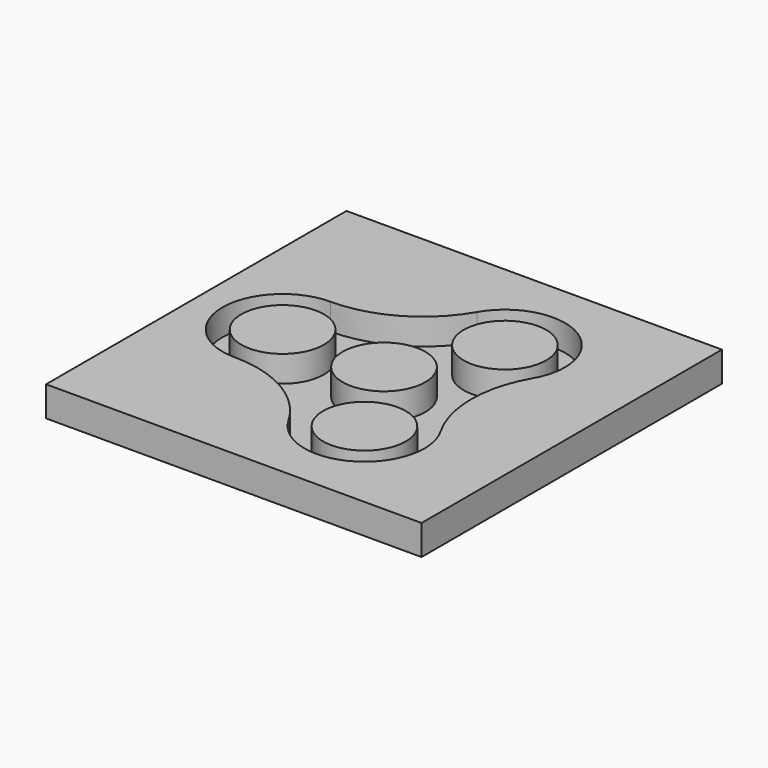
from build123d import *

# Parameters (mm, degrees)
F0_W     = 100
F0_H     = 100
F1_DEPTH = 7
F0_R     = 11
F2_DEPTH = 7
F3_R     = 3.49999
F5_W     = 100
F5_H     = 100
F6_DEPTH = 1
F7_R     = 11
F8_DEPTH = 7


# Not quite as in the source:
# - a fillet or chamfer is up to 0.001 mm smaller than in the source, because OpenCascade refuses the exact size


with BuildPart() as f1:
    # F0 (on Top) → F1 (new body)
    with BuildSketch(Plane.XY):
        Rectangle(F0_W, F0_H)
        with BuildLine():
            ThreePointArc((-27, 16), (-11.6173140978, 20.1217782649), (-0.3564064606, 31.3826859022))
            ThreePointArc((-0.3564064606, 31.3826859022), (17.6411047216, 38.8374991228), (29.5, 23.3826859022))
            ThreePointArc((29.5, 23.3826859022), (28.9548132206, 19.2415811805), (27.3564064606, 15.3826859022))
            ThreePointArc((27.3564064606, 15.3826859022), (23.2346281956, 0), (27.3564064606, -15.3826859022))
            ThreePointArc((27.3564064606, -15.3826859022), (28.9548132206, -19.2415811805), (29.5, -23.3826859022))
            ThreePointArc((29.5, -23.3826859022), (17.6411047216, -38.8374991228), (-0.3564064606, -31.3826859022))
            ThreePointArc((-0.3564064606, -31.3826859022), (-11.6173140978, -20.1217782649), (-27, -16))
            ThreePointArc((-27, -16), (-43, 0), (-27, 16))
        make_face(mode=Mode.SUBTRACT)
    extrude(amount=F1_DEPTH)


with BuildPart() as f2:
    # F0 (on Top) → F2 (new body)
    with BuildSketch(Plane.XY):
        with BuildLine():
            ThreePointArc((-16, 0), (-15.3622914957, 4.472135955), (-13.5, 8.5877820187))
            ThreePointArc((-13.5, 8.5877820187), (-19.299497169, 14.0250581514), (-27, 16))
            ThreePointArc((-27, 16), (-43, 0), (-27, -16))
            ThreePointArc((-27, -16), (-19.299497169, -14.0250581514), (-13.5, -8.5877820187))
            ThreePointArc((-13.5, -8.5877820187), (-15.3622914957, -4.472135955), (-16, 0))
        make_face()
        with Locations((-27, 0)):
            Circle(F0_R, mode=Mode.SUBTRACT)
        with BuildLine():
            ThreePointArc((-0.3564064606, 31.3826859022), (-2.4963080642, 23.7263839043), (-0.6872373903, 15.9852339604))
            ThreePointArc((-0.6872373903, 15.9852339604), (3.8081625511, 15.5402026365), (8.0000002665, 13.8564063067))
            ThreePointArc((8.0000002665, 13.8564063067), (11.5541292005, 11.068066607), (14.1872373903, 7.3974519418))
            ThreePointArc((14.1872373903, 7.3974519418), (21.7958052331, 9.7013257529), (27.3564064606, 15.3826859022))
            ThreePointArc((27.3564064606, 15.3826859022), (28.9548132206, 19.2415811805), (29.5, 23.3826859022))
            ThreePointArc((29.5, 23.3826859022), (17.6411047216, 38.8374991228), (-0.3564064606, 31.3826859022))
        make_face()
        with BuildLine():
            ThreePointArc((24.5, 23.3826859022), (19.0000001332, 13.8564065375), (8.0000002665, 13.8564063067))
            ThreePointArc((8.0000002665, 13.8564063067), (7.9999998668, 32.9089652669), (24.5, 23.3826859022))
        make_face(mode=Mode.SUBTRACT)
        with BuildLine():
            ThreePointArc((-0.6872373903, 15.9852339604), (1.9458710013, 12.3146190845), (5.5000002388, 9.5262793037))
            ThreePointArc((5.5000002388, 9.5262793037), (9.6918377323, 7.8424831962), (14.1872373903, 7.3974519418))
            ThreePointArc((14.1872373903, 7.3974519418), (11.5541292005, 11.068066607), (8.0000002665, 13.8564063067))
            ThreePointArc((8.0000002665, 13.8564063067), (3.8081625511, 15.5402026365), (-0.6872373903, 15.9852339604))
        make_face()
        with BuildLine():
            ThreePointArc((27.3564064606, -15.3826859022), (21.7958052331, -9.7013257529), (14.1872373903, -7.3974519418))
            ThreePointArc((14.1872373903, -7.3974519418), (11.5541290581, -11.0680667557), (7.99999991, -13.8564065125))
            ThreePointArc((7.99999991, -13.8564065125), (3.8081623512, -15.5402026855), (-0.6872373903, -15.9852339604))
            ThreePointArc((-0.6872373903, -15.9852339604), (-2.4963080642, -23.7263839043), (-0.3564064606, -31.3826859022))
            ThreePointArc((-0.3564064606, -31.3826859022), (17.6411047216, -38.8374991228), (29.5, -23.3826859022))
            ThreePointArc((29.5, -23.3826859022), (28.9548132206, -19.2415811805), (27.3564064606, -15.3826859022))
        make_face()
        with BuildLine():
            ThreePointArc((24.5, -23.3826859022), (8.000000045, -32.9089653698), (7.99999991, -13.8564065125))
            ThreePointArc((7.99999991, -13.8564065125), (18.999999955, -13.8564064346), (24.5, -23.3826859022))
        make_face(mode=Mode.SUBTRACT)
        with BuildLine():
            ThreePointArc((14.1872373903, -7.3974519418), (9.6918376596, -7.842483214), (5.5000001093, -9.5262793785))
            ThreePointArc((5.5000001093, -9.5262793785), (1.9458709496, -12.3146191385), (-0.6872373903, -15.9852339604))
            ThreePointArc((-0.6872373903, -15.9852339604), (3.8081623512, -15.5402026855), (7.99999991, -13.8564065125))
            ThreePointArc((7.99999991, -13.8564065125), (11.5541290581, -11.0680667557), (14.1872373903, -7.3974519418))
        make_face()
        with BuildLine():
            ThreePointArc((-0.3564064606, -31.3826859022), (-2.4963080642, -23.7263839043), (-0.6872373903, -15.9852339604))
            ThreePointArc((-0.6872373903, -15.9852339604), (-8, -13.8564064606), (-13.5, -8.5877820187))
            ThreePointArc((-13.5, -8.5877820187), (-19.299497169, -14.0250581514), (-27, -16))
            ThreePointArc((-27, -16), (-11.6173140978, -20.1217782649), (-0.3564064606, -31.3826859022))
        make_face()
        with BuildLine():
            ThreePointArc((5.5000002388, 9.5262793037), (9.5262795106, 5.4999998806), (11, 0))
            ThreePointArc((11, 0), (9.5262794732, -5.4999999453), (5.5000001093, -9.5262793785))
            ThreePointArc((5.5000001093, -9.5262793785), (9.6918376596, -7.842483214), (14.1872373903, -7.3974519418))
            ThreePointArc((14.1872373903, -7.3974519418), (15.5402026731, -3.8081624017), (16, 0))
            ThreePointArc((16, 0), (15.5402026731, 3.8081624017), (14.1872373903, 7.3974519418))
            ThreePointArc((14.1872373903, 7.3974519418), (9.6918377323, 7.8424831962), (5.5000002388, 9.5262793037))
        make_face()
        with BuildLine():
            ThreePointArc((-0.6872373903, -15.9852339604), (1.9458709496, -12.3146191385), (5.5000001093, -9.5262793785))
            ThreePointArc((5.5000001093, -9.5262793785), (-5.4999999453, -9.5262794732), (-11, 0))
            ThreePointArc((-11, 0), (-11.6377085043, -4.472135955), (-13.5, -8.5877820187))
            ThreePointArc((-13.5, -8.5877820187), (-8, -13.8564064606), (-0.6872373903, -15.9852339604))
        make_face()
        with BuildLine():
            ThreePointArc((-13.5, -8.5877820187), (-11.6377085043, -4.472135955), (-11, 0))
            ThreePointArc((-11, 0), (-11.6377085043, 4.472135955), (-13.5, 8.5877820187))
            ThreePointArc((-13.5, 8.5877820187), (-15.3622914957, 4.472135955), (-16, 0))
            ThreePointArc((-16, 0), (-15.3622914957, -4.472135955), (-13.5, -8.5877820187))
        make_face()
        with BuildLine():
            ThreePointArc((-11, 0), (-5.4999998806, 9.5262795106), (5.5000002388, 9.5262793037))
            ThreePointArc((5.5000002388, 9.5262793037), (1.9458710013, 12.3146190845), (-0.6872373903, 15.9852339604))
            ThreePointArc((-0.6872373903, 15.9852339604), (-8, 13.8564064606), (-13.5, 8.5877820187))
            ThreePointArc((-13.5, 8.5877820187), (-11.6377085043, 4.472135955), (-11, 0))
        make_face()
        with BuildLine():
            ThreePointArc((-13.5, 8.5877820187), (-8, 13.8564064606), (-0.6872373903, 15.9852339604))
            ThreePointArc((-0.6872373903, 15.9852339604), (-2.4963080642, 23.7263839043), (-0.3564064606, 31.3826859022))
            ThreePointArc((-0.3564064606, 31.3826859022), (-11.6173140978, 20.1217782649), (-27, 16))
            ThreePointArc((-27, 16), (-19.299497169, 14.0250581514), (-13.5, 8.5877820187))
        make_face()
        with BuildLine():
            ThreePointArc((27.3564064606, 15.3826859022), (21.7958052331, 9.7013257529), (14.1872373903, 7.3974519418))
            ThreePointArc((14.1872373903, 7.3974519418), (15.5402026731, 3.8081624017), (16, 0))
            ThreePointArc((16, 0), (15.5402026731, -3.8081624017), (14.1872373903, -7.3974519418))
            ThreePointArc((14.1872373903, -7.3974519418), (21.7958052331, -9.7013257529), (27.3564064606, -15.3826859022))
            ThreePointArc((27.3564064606, -15.3826859022), (23.2346281956, 0), (27.3564064606, 15.3826859022))
        make_face()
    extrude(amount=F2_DEPTH)

    # F3 (radius 3.5 in the source; OpenCascade refuses exactly that, so slightly less here)
    f3_edges = [f2.edges().sort_by_distance(p)[0] for p in [
        (21.5, 37.239092, 7),
        (21.5, 37.239092, 0),
    ]]
    fillet(f3_edges, radius=F3_R)


with BuildPart() as f1_1:
    add(f1.part)

    # F4: cut F2
    add(f2.part, mode=Mode.SUBTRACT)

    # F5 (on Top) → F6 (join)
    with BuildSketch(Plane.XY):
        Rectangle(F5_W, F5_H)
    extrude(amount=-F6_DEPTH)

    # F7 (on face) → F8 (join)
    with BuildSketch(Plane.XY):
        Circle(F7_R)
        with Locations((13.5, 23.3826859022)):
            Circle(F7_R)
        with Locations((-27, 0)):
            Circle(F7_R)
        with Locations((13.5, -23.3826859022)):
            Circle(F7_R)
    extrude(amount=F8_DEPTH)


solid = f1_1.part
